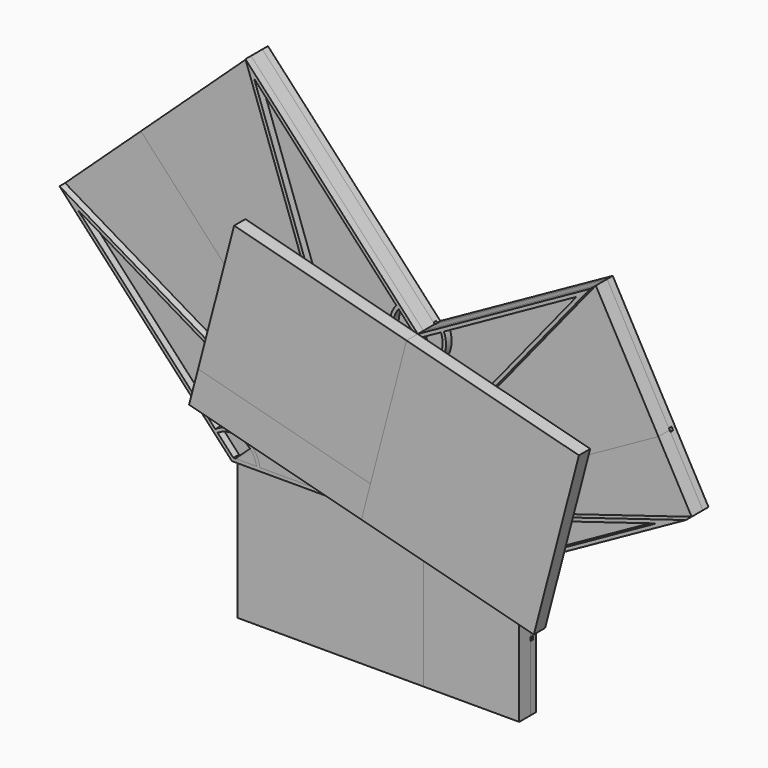
from build123d import *

# Parameters (mm, degrees)
F0_W      = 43.18
F0_H      = 63.5
F1_DEPTH  = 3.175
F5_DEPTH  = 1.524
F6_DEPTH  = 9.525
F7_DEPTH  = 6.35
F8_DEPTH  = 6.35
F9_DEPTH  = 6.35
F13_DEPTH = 6.35
F15_DEPTH = 6.35
F17_DEPTH = 6.35
F19_DEPTH = 3.175
F21_DEPTH = 3.175
F23_DEPTH = 3.175
F25_DEPTH = 3.175


# Not quite as in the source:
# - the program builds the solid bodies; features that only make, move or delete a surface that nothing else refers to are left out


with BuildPart() as f1:
    # F0 (on Front) → F1 (new body)
    with BuildSketch(Plane.XZ):
        Polygon((-63.5, 0), (0, 0), (20.32, 77.7090573872), (-29.3511111111, 31.6592456022), align=None)
        Polygon((20.32, 77.7090573872), (0, 0), (20.32, 0), (63.5, 0), (48.5191836735, 26.960285216), align=None)
        Polygon((-29.3511111111, 31.6592456022), (20.32, 77.7090573872), (-57.3890573872, 161.5290573872), (-107.0601684983, 115.4792456022), align=None)
        Polygon((-141.2090573872, 83.82), (-63.5, 0), (-29.3511111111, 31.6592456022), (-107.0601684983, 115.4792456022), align=None)
        Polygon((98.0290573872, 120.8890573872), (20.32, 77.7090573872), (48.5191836735, 26.960285216), (126.2282410606, 70.140285216), align=None)
        Polygon((126.2282410606, 70.140285216), (48.5191836735, 26.960285216), (63.5, 0), (141.2090573872, 43.18), align=None)
        with Locations((41.91, -31.75)):
            Rectangle(F0_W, F0_H)
        Polygon((20.32, 0), (0, 0), (-63.5, 0), (-63.5, -63.5), (20.32, -63.5), align=None)
    extrude(amount=-F1_DEPTH)

    # F2 (on face) + F3 (on face) + F4 (on face) → F5 (cut)
    with BuildSketch(Plane.XZ):
        with BuildLine():
            Line((19.7446540943, 77.1756573872), (20.32, 77.7090573872))
            Line((20.32, 77.7090573872), (20.7010732622, 77.0232573872))
            Line((20.7010732622, 77.0232573872), (20.8380603826, 77.1502573872))
            ThreePointArc((20.8380603826, 77.1502573872), (21.0725065771, 77.5891497084), (20.9860776347, 78.0791716729))
            ThreePointArc((20.9860776347, 78.0791716729), (20.4399076788, 78.4615639642), (19.8019396174, 78.2678573872))
            ThreePointArc((19.8019396174, 78.2678573872), (19.5674934229, 77.8289650659), (19.6539223653, 77.3389431014))
            Line((19.6539223653, 77.3389431014), (19.7446540943, 77.1756573872))
        make_face()
        with BuildLine():
            Line((-62.6780772776, 0.762), (19.7446540943, 77.1756573872))
            Line((19.7446540943, 77.1756573872), (19.6539223653, 77.3389431014))
            ThreePointArc((19.6539223653, 77.3389431014), (19.5674934229, 77.8289650659), (19.8019396174, 78.2678573872))
            Line((19.8019396174, 78.2678573872), (-64.0180603826, 0.5588))
            ThreePointArc((-64.0180603826, 0.5588), (-63.7782430592, 0.7093833942), (-63.5, 0.762))
            Line((-63.5, 0.762), (-62.6780772776, 0.762))
        make_face()
        with BuildLine():
            Line((20.8380603826, 77.1502573872), (20.7010732622, 77.0232573872))
            Line((20.7010732622, 77.0232573872), (63.0765852642, 0.762))
            Line((63.0765852642, 0.762), (63.5, 0.762))
            ThreePointArc((63.5, 0.762), (63.8864045253, 0.6567614048), (64.1660776347, 0.3701142857))
            Line((64.1660776347, 0.3701142857), (20.9860776347, 78.0791716729))
            ThreePointArc((20.9860776347, 78.0791716729), (21.0725065771, 77.5891497084), (20.8380603826, 77.1502573872))
        make_face()
        with BuildLine():
            Line((-63.5, 0), (-62.6780772776, 0.762))
            Line((-62.6780772776, 0.762), (-63.5, 0.762))
            ThreePointArc((-63.5, 0.762), (-63.7782430592, 0.7093833942), (-64.0180603826, 0.5588))
            ThreePointArc((-64.0180603826, 0.5588), (-64.2093833942, -0.2782430592), (-63.5, -0.762))
            ThreePointArc((-63.5, -0.762), (-63.2217569408, -0.7093833942), (-62.9819396174, -0.5588))
            Line((-62.9819396174, -0.5588), (-62.3791962877, 0))
            Line((-62.3791962877, 0), (-63.5, 0))
        make_face()
        with BuildLine():
            Line((63.5, 0.762), (63.0765852642, 0.762))
            Line((63.0765852642, 0.762), (63.5, 0))
            Line((63.5, 0), (62.6282637793, 0))
            Line((62.6282637793, 0), (62.8339223653, -0.3701142857))
            ThreePointArc((62.8339223653, -0.3701142857), (63.1135954747, -0.6567614048), (63.5, -0.762))
            ThreePointArc((63.5, -0.762), (64.1567614048, -0.3864045253), (64.1660776347, 0.3701142857))
            ThreePointArc((64.1660776347, 0.3701142857), (63.8864045253, 0.6567614048), (63.5, 0.762))
        make_face()
        with BuildLine():
            Line((62.6282637793, 0), (-62.3791962877, 0))
            Line((-62.3791962877, 0), (-62.9819396174, -0.5588))
            ThreePointArc((-62.9819396174, -0.5588), (-63.2217569408, -0.7093833942), (-63.5, -0.762))
            Line((-63.5, -0.762), (63.5, -0.762))
            ThreePointArc((63.5, -0.762), (63.1135954747, -0.6567614048), (62.8339223653, -0.3701142857))
            Line((62.8339223653, -0.3701142857), (62.6282637793, 0))
        make_face()
    with BuildSketch(Plane.XZ):
        Polygon((4.9939852947, 16.0862518798), (4.2567724462, 16.2790243259), (4.064, 15.5418114774), (4.8012128485, 15.3490390313), align=None)
        with BuildLine():
            Line((3.5195595977, 16.4717967721), (4.2567724462, 16.2790243259))
            Line((4.2567724462, 16.2790243259), (4.9939852947, 16.0862518798))
            Line((4.9939852947, 16.0862518798), (21.0572128485, 77.516284941))
            ThreePointArc((21.0572128485, 77.516284941), (20.5127724462, 78.4462702357), (19.5827871515, 77.9018298333))
            Line((19.5827871515, 77.9018298333), (3.5195595977, 16.4717967721))
        make_face()
        Polygon((4.064, 15.5418114774), (4.2567724462, 16.2790243259), (3.5195595977, 16.4717967721), (3.3267871515, 15.7345839236), align=None)
        Polygon((4.8012128485, 15.3490390313), (4.064, 15.5418114774), (3.8712275538, 14.8045986289), (4.6084404023, 14.6118261828), align=None)
        Polygon((3.8712275538, 14.8045986289), (4.064, 15.5418114774), (3.3267871515, 15.7345839236), (3.1340147053, 14.9973710751), align=None)
        with BuildLine():
            Line((63.6927724462, 0.7372128485), (4.9939852947, 16.0862518798))
            Line((4.9939852947, 16.0862518798), (4.8012128485, 15.3490390313))
            Line((4.8012128485, 15.3490390313), (4.6084404023, 14.6118261828))
            Line((4.6084404023, 14.6118261828), (63.3072275538, -0.7372128485))
            ThreePointArc((63.3072275538, -0.7372128485), (64.2372128485, -0.1927724462), (63.6927724462, 0.7372128485))
        make_face()
        with BuildLine():
            Line((3.3267871515, 15.7345839236), (3.5195595977, 16.4717967721))
            Line((3.5195595977, 16.4717967721), (-73.452284941, 36.5990243259))
            ThreePointArc((-73.452284941, 36.5990243259), (-74.3822702357, 36.0545839236), (-73.8378298333, 35.1245986289))
            Line((-73.8378298333, 35.1245986289), (3.1340147053, 14.9973710751))
            Line((3.1340147053, 14.9973710751), (3.3267871515, 15.7345839236))
        make_face()
        with BuildLine():
            Line((4.6084404023, 14.6118261828), (3.8712275538, 14.8045986289))
            Line((3.8712275538, 14.8045986289), (0.1927724462, 0.7372128485))
            ThreePointArc((0.1927724462, 0.7372128485), (0.6031320767, 0.4656991497), (0.762, 0))
            Line((0.762, 0), (0.762, -0.0979798193))
            Line((0.762, -0.0979798193), (4.6084404023, 14.6118261828))
        make_face()
        with BuildLine():
            Line((0.1927724462, 0.7372128485), (3.8712275538, 14.8045986289))
            Line((3.8712275538, 14.8045986289), (3.1340147053, 14.9973710751))
            Line((3.1340147053, 14.9973710751), (-0.7372128485, 0.1927724462))
            ThreePointArc((-0.7372128485, 0.1927724462), (-0.3849775004, 0.6575989083), (0.1927724462, 0.7372128485))
        make_face()
        with BuildLine():
            ThreePointArc((0.762, 0), (0.6031320767, 0.4656991497), (0.1927724462, 0.7372128485))
            Line((0.1927724462, 0.7372128485), (0, 0))
            Line((0, 0), (0, -0.762))
            ThreePointArc((0, -0.762), (0.4656991497, -0.6031320767), (0.7372128485, -0.1927724462))
            Line((0.7372128485, -0.1927724462), (0.762, -0.0979798193))
            Line((0.762, -0.0979798193), (0.762, 0))
        make_face()
        with BuildLine():
            Line((0, 0), (0.1927724462, 0.7372128485))
            ThreePointArc((0.1927724462, 0.7372128485), (-0.3849775004, 0.6575989083), (-0.7372128485, 0.1927724462))
            ThreePointArc((-0.7372128485, 0.1927724462), (-0.7557778081, 0.0971797547), (-0.762, 0))
            ThreePointArc((-0.762, 0), (-0.5388153673, -0.5388153673), (0, -0.762))
            Line((0, -0.762), (0, 0))
        make_face()
        with BuildLine():
            Line((0.762, -16.0161328704), (0.762, -0.0979798193))
            Line((0.762, -0.0979798193), (0.7372128485, -0.1927724462))
            ThreePointArc((0.7372128485, -0.1927724462), (0.4656991497, -0.6031320767), (0, -0.762))
            Line((0, -0.762), (0, -15.8168788771))
            Line((0, -15.8168788771), (0.762, -16.0161328704))
        make_face()
        with BuildLine():
            Line((0, -15.8168788771), (0, -0.762))
            ThreePointArc((0, -0.762), (-0.5388153673, -0.5388153673), (-0.762, 0))
            Line((-0.762, 0), (-0.762, -15.6176248838))
            Line((-0.762, -15.6176248838), (0, -15.8168788771))
        make_face()
        with BuildLine():
            Line((73.8378298333, -35.1245986289), (0.762, -16.0161328704))
            Line((0.762, -16.0161328704), (0.762, -16.803753435))
            Line((0.762, -16.803753435), (0.762, -17.5913739996))
            Line((0.762, -17.5913739996), (73.452284941, -36.5990243259))
            ThreePointArc((73.452284941, -36.5990243259), (74.3822702357, -36.0545839236), (73.8378298333, -35.1245986289))
        make_face()
        Polygon((0.762, -16.803753435), (0.762, -16.0161328704), (0, -15.8168788771), (0, -16.6044994417), align=None)
        Polygon((0, -16.6044994417), (0, -15.8168788771), (-0.762, -15.6176248838), (-0.762, -16.4052454484), align=None)
        with BuildLine():
            Line((-0.762, -16.4052454484), (-0.762, -15.6176248838))
            Line((-0.762, -15.6176248838), (-63.3072275538, 0.7372128485))
            ThreePointArc((-63.3072275538, 0.7372128485), (-64.2372128485, 0.1927724462), (-63.6927724462, -0.7372128485))
            Line((-63.6927724462, -0.7372128485), (-0.762, -17.192866013))
            Line((-0.762, -17.192866013), (-0.762, -16.4052454484))
        make_face()
        Polygon((0.762, -17.5913739996), (0.762, -16.803753435), (0, -16.6044994417), (0, -17.3921200063), align=None)
        Polygon((0, -17.3921200063), (0, -16.6044994417), (-0.762, -16.4052454484), (-0.762, -17.192866013), align=None)
        with BuildLine():
            Line((0.762, -63.5), (0.762, -17.5913739996))
            Line((0.762, -17.5913739996), (0, -17.3921200063))
            Line((0, -17.3921200063), (-0.762, -17.192866013))
            Line((-0.762, -17.192866013), (-0.762, -63.5))
            ThreePointArc((-0.762, -63.5), (0, -64.262), (0.762, -63.5))
        make_face()
    with BuildSketch(Plane.XZ):
        with BuildLine():
            Line((-0.5180603826, 0.5588), (0, 0))
            Line((0, 0), (0.6660776347, 0.3701142857))
            ThreePointArc((0.6660776347, 0.3701142857), (0.6168900363, 0.4473149708), (0.5588, 0.5180603826))
            Line((0.5588, 0.5180603826), (0.1524, 0.9564191678))
            Line((0.1524, 0.9564191678), (-0.3701142857, 0.6660776347))
            ThreePointArc((-0.3701142857, 0.6660776347), (-0.4473149708, 0.6168900363), (-0.5180603826, 0.5588))
        make_face()
        with BuildLine():
            Line((0.6660776347, 0.3701142857), (0, 0))
            Line((0, 0), (-0.5180603826, 0.5588))
            ThreePointArc((-0.5180603826, 0.5588), (-0.7614552789, 0.0288072597), (-0.5588, -0.5180603826))
            ThreePointArc((-0.5588, -0.5180603826), (-0.1199076788, -0.7525065771), (0.3701142857, -0.6660776347))
            ThreePointArc((0.3701142857, -0.6660776347), (0.7326983336, -0.2092776911), (0.6660776347, 0.3701142857))
        make_face()
        with BuildLine():
            ThreePointArc((0.5588, 0.5180603826), (0.6168900363, 0.4473149708), (0.6660776347, 0.3701142857))
            Line((0.6660776347, 0.3701142857), (19.558, 10.8676448846))
            Line((19.558, 10.8676448846), (19.558, 11.7393811053))
            Line((19.558, 11.7393811053), (0.1524, 0.9564191678))
            Line((0.1524, 0.9564191678), (0.5588, 0.5180603826))
        make_face()
        with BuildLine():
            Line((19.558, 10.8676448846), (0.6660776347, 0.3701142857))
            ThreePointArc((0.6660776347, 0.3701142857), (0.7326983336, -0.2092776911), (0.3701142857, -0.6660776347))
            Line((0.3701142857, -0.6660776347), (19.558, 9.9959086639))
            Line((19.558, 9.9959086639), (19.558, 10.8676448846))
        make_face()
        with BuildLine():
            ThreePointArc((-0.5588, -0.5180603826), (-0.7614552789, 0.0288072597), (-0.5180603826, 0.5588))
            ThreePointArc((-0.5180603826, 0.5588), (-0.4473149708, 0.6168900363), (-0.3701142857, 0.6660776347))
            Line((-0.3701142857, 0.6660776347), (0.1524, 0.9564191678))
            Line((0.1524, 0.9564191678), (-106.5013684983, 115.9973059848))
            ThreePointArc((-106.5013684983, 115.9973059848), (-107.5782288808, 116.0380456022), (-107.6189684983, 114.9611852196))
            Line((-107.6189684983, 114.9611852196), (-0.5588, -0.5180603826))
        make_face()
        Polygon((19.558, 11.7393811053), (19.558, 10.8676448846), (20.32, 11.2910596204), (20.32, 12.162795841), align=None)
        Polygon((20.32, 11.2910596204), (19.558, 10.8676448846), (19.558, 9.9959086639), (20.32, 10.4193233997), align=None)
        Polygon((20.32, 12.162795841), (20.32, 11.2910596204), (21.082, 11.7144743561), (21.082, 12.5862105768), align=None)
        Polygon((21.082, 11.7144743561), (20.32, 11.2910596204), (20.32, 10.4193233997), (21.082, 10.8427381354), align=None)
        with BuildLine():
            Line((20.32, 10.4193233997), (19.558, 9.9959086639))
            Line((19.558, 9.9959086639), (19.558, -63.5))
            ThreePointArc((19.558, -63.5), (20.32, -64.262), (21.082, -63.5))
            Line((21.082, -63.5), (21.082, 10.8427381354))
            Line((21.082, 10.8427381354), (20.32, 10.4193233997))
        make_face()
        with BuildLine():
            Line((19.558, 77.7090573872), (19.558, 11.7393811053))
            Line((19.558, 11.7393811053), (20.32, 12.162795841))
            Line((20.32, 12.162795841), (21.082, 12.5862105768))
            Line((21.082, 12.5862105768), (21.082, 77.7090573872))
            ThreePointArc((21.082, 77.7090573872), (20.32, 78.4710573872), (19.558, 77.7090573872))
        make_face()
        with BuildLine():
            Line((21.082, 12.5862105768), (21.082, 11.7144743561))
            Line((21.082, 11.7144743561), (21.082, 10.8427381354))
            Line((21.082, 10.8427381354), (126.5983553463, 69.4742075812))
            ThreePointArc((126.5983553463, 69.4742075812), (126.8943186954, 70.5103995017), (125.8581267749, 70.8063628507))
            Line((125.8581267749, 70.8063628507), (21.082, 12.5862105768))
        make_face()
    extrude(amount=-F5_DEPTH, mode=Mode.SUBTRACT)


with BuildPart() as f6:
    # F0 (on Front) → F6 (new body)
    with BuildSketch(Plane.XZ):
        Polygon((-63.5, 0), (0, 0), (20.32, 77.7090573872), (-29.3511111111, 31.6592456022), align=None)
        Polygon((20.32, 77.7090573872), (0, 0), (20.32, 0), (63.5, 0), (48.5191836735, 26.960285216), align=None)
    extrude(amount=F6_DEPTH)


with BuildPart() as f7:
    # F0 (on Front) → F7 (new body)
    with BuildSketch(Plane.XZ):
        Polygon((-141.2090573872, 83.82), (-63.5, 0), (-29.3511111111, 31.6592456022), (-107.0601684983, 115.4792456022), align=None)
    extrude(amount=F7_DEPTH)


with BuildPart() as f7b:
    # F0 (on Front) → F7, piece 2 (new body)
    with BuildSketch(Plane.XZ):
        Polygon((20.32, 0), (0, 0), (-63.5, 0), (-63.5, -63.5), (20.32, -63.5), align=None)
    extrude(amount=F7_DEPTH)


with BuildPart() as f8:
    # F0 (on Front) → F8 (new body)
    with BuildSketch(Plane.XZ):
        Polygon((126.2282410606, 70.140285216), (48.5191836735, 26.960285216), (63.5, 0), (141.2090573872, 43.18), align=None)
    extrude(amount=F8_DEPTH)


with BuildPart() as f8b:
    # F0 (on Front) → F8, piece 2 (new body)
    with BuildSketch(Plane.XZ):
        with Locations((41.91, -31.75)):
            Rectangle(F0_W, F0_H)
    extrude(amount=F8_DEPTH)


with BuildPart() as f9:
    # F0 (on Front) → F9 (new body)
    with BuildSketch(Plane.XZ):
        Polygon((-29.3511111111, 31.6592456022), (20.32, 77.7090573872), (-57.3890573872, 161.5290573872), (-107.0601684983, 115.4792456022), align=None)
    extrude(amount=F9_DEPTH)


with BuildPart() as f9b:
    # F0 (on Front) → F9, piece 2 (new body)
    with BuildSketch(Plane.XZ):
        Polygon((98.0290573872, 120.8890573872), (20.32, 77.7090573872), (48.5191836735, 26.960285216), (126.2282410606, 70.140285216), align=None)
    extrude(amount=F9_DEPTH)


with BuildPart() as f13:
    # F12 (on face) → F13 (new body)
    with BuildSketch(Plane.XZ.offset(9.525)):
        Polygon((98.0290573872, 57.3890573872), (20.32, 77.7090573872), (4.064, 15.5418114774), (0, 0), (77.7090573872, -20.32), align=None)
    extrude(amount=F13_DEPTH)


with BuildPart() as f15:
    # F14 (on face) → F15 (new body)
    with BuildSketch(Plane.XZ.offset(9.525)):
        Polygon((-73.6450573872, 35.8618114774), (4.064, 15.5418114774), (20.32, 77.7090573872), (-57.3890573872, 98.0290573872), align=None)
    extrude(amount=F15_DEPTH)


with BuildPart() as f17:
    # F16 (on face) → F17 (new body)
    with BuildSketch(Plane.XZ.offset(9.525)):
        Polygon((0, 0), (4.064, 15.5418114774), (-73.6450573872, 35.8618114774), (-77.7090573872, 20.32), align=None)
    extrude(amount=F17_DEPTH)


with BuildPart() as f19:
    # F18 (on face) → F19 (new body)
    with BuildSketch(Plane.XZ.offset(9.525)):
        Polygon((-63.5, 0), (0, 0), (-141.2090573872, 83.82), align=None)
        with BuildLine():
            Line((-52.4283966834, 1.524), (-62.8347101343, 1.524))
            Line((-62.8347101343, 1.524), (-69.9096428477, 9.1552965307))
            ThreePointArc((-69.9096428477, 9.1552965307), (-59.0286869336, 10.2425746501), (-52.4283966834, 1.524))
        make_face(mode=Mode.SUBTRACT)
        with BuildLine():
            Line((-70.9543470357, 10.282154943), (-132.9338950323, 77.1356967019))
            Line((-132.9338950323, 77.1356967019), (-5.5531217238, 1.524))
            Line((-5.5531217238, 1.524), (-50.8917715757, 1.524))
            ThreePointArc((-50.8917715757, 1.524), (-58.4189624245, 11.6392893751), (-70.9543470357, 10.282154943))
        make_face(mode=Mode.SUBTRACT)
    extrude(amount=-F19_DEPTH)


with BuildPart() as f21:
    # F20 (on face) → F21 (new body)
    with BuildSketch(Plane.XZ.offset(9.525)):
        Polygon((141.2090573872, 43.18), (0, 0), (63.5, 0), align=None)
        with BuildLine():
            ThreePointArc((52.4283966834, 1.524), (60.6961559845, 10.8185689782), (72.43765509, 6.7097911661))
            Line((72.43765509, 6.7097911661), (63.1050255548, 1.524))
            Line((63.1050255548, 1.524), (52.4283966834, 1.524))
        make_face(mode=Mode.SUBTRACT)
        with BuildLine():
            Line((50.8917715757, 1.524), (10.1955021516, 1.524))
            Line((10.1955021516, 1.524), (127.8538317039, 37.5024759142))
            Line((127.8538317039, 37.5024759142), (73.7808461887, 7.4561519327))
            ThreePointArc((73.7808461887, 7.4561519327), (60.3138136188, 12.2938283844), (50.8917715757, 1.524))
        make_face(mode=Mode.SUBTRACT)
    extrude(amount=-F21_DEPTH)


with BuildPart() as f23:
    # F22 (on face) → F23 (new body)
    with BuildSketch(Plane.XZ.offset(9.525)):
        Polygon((20.32, 77.7090573872), (0, 0), (98.0290573872, 120.8890573872), align=None)
        with BuildLine():
            Line((18.9935069906, 66.6120581398), (21.6296321213, 76.693298251))
            Line((21.6296321213, 76.693298251), (30.7381122328, 81.7545380143))
            ThreePointArc((30.7381122328, 81.7545380143), (29.1510848265, 70.8596109287), (18.9935069906, 66.6120581398))
        make_face(mode=Mode.SUBTRACT)
        with BuildLine():
            Line((91.8845396074, 115.7313075546), (3.2588042137, 6.4383907648))
            Line((3.2588042137, 6.4383907648), (18.6047681706, 65.1254180181))
            ThreePointArc((18.6047681706, 65.1254180181), (30.3553236665, 69.9255955026), (32.0813033316, 82.5008987809))
            Line((32.0813033316, 82.5008987809), (91.8845396074, 115.7313075546))
        make_face(mode=Mode.SUBTRACT)
    extrude(amount=-F23_DEPTH)


with BuildPart() as f25:
    # F24 (on face) → F25 (new body)
    with BuildSketch(Plane.XZ.offset(9.525)):
        Polygon((-57.3890573872, 161.5290573872), (0, 0), (20.32, 77.7090573872), align=None)
        with BuildLine():
            Line((-0.2217168917, 5.1762348747), (-53.4755673695, 155.0662080081))
            Line((-53.4755673695, 155.0662080081), (10.6304529643, 85.9189707998))
            ThreePointArc((10.6304529643, 85.9189707998), (8.0020686996, 74.6173639226), (15.6559167765, 65.8965078027))
            Line((15.6559167765, 65.8965078027), (-0.2217168917, 5.1762348747))
        make_face(mode=Mode.SUBTRACT)
        with BuildLine():
            ThreePointArc((16.0446555966, 67.3831479244), (9.4802204556, 74.9883671384), (11.6751571523, 84.7921123875))
            Line((11.6751571523, 84.7921123875), (18.6341119192, 77.2859141633))
            Line((18.6341119192, 77.2859141633), (16.0446555966, 67.3831479244))
        make_face(mode=Mode.SUBTRACT)
    extrude(amount=-F25_DEPTH)


solid = Compound([f1.part, f6.part, f7.part, f7b.part, f8.part, f8b.part, f9.part, f9b.part, f13.part, f15.part, f17.part, f19.part, f21.part, f23.part, f25.part])
